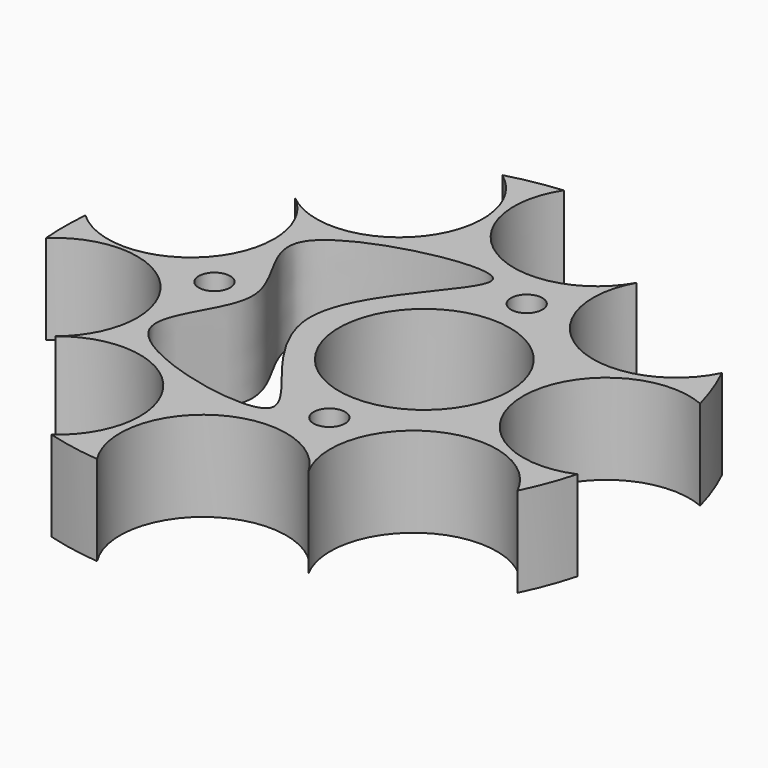
from build123d import *

# Parameters (mm, degrees)
F0_R     = 1.75
F0_R_2   = 9.5
F1_DEPTH = 10


with BuildPart() as f1:
    # F0 (on Top) → F1 (new body)
    with BuildSketch(Plane.XY):
        with BuildLine():
            ThreePointArc((31.353928612, -8.5545987979), (18.4999848113, -0.0237061853), (31.3757496158, 8.4742159547))
            ThreePointArc((31.3757496158, 8.4742159547), (30.4507046637, 11.3580185545), (29.2612387482, 14.1431929536))
            ThreePointArc((29.2612387482, 14.1431929536), (16.6372633011, 10.0158268124), (12.9009909928, 22.7610289132))
            ThreePointArc((12.9009909928, 22.7610289132), (0.046675345, 19.4194010798), (-2.8971318292, 32.3706136359))
            ThreePointArc((-2.8971318292, 32.3706136359), (-5.8977553578, 31.9603892614), (-8.8471652882, 31.2726344647))
            ThreePointArc((-8.8471652882, 31.2726344647), (-6.0434782071, 27.9889108187), (-5.0357213297, 23.7903481709))
            ThreePointArc((-5.0357213297, 23.7903481709), (-10.3432199295, 15.4226015979), (-20.1750040777, 16.6574070724))
            ThreePointArc((-20.1750040777, 16.6574070724), (-17.6965402546, 13.4669673747), (-16.8142868283, 9.5244659761))
            ThreePointArc((-16.8142868283, 9.5244659761), (-22.3815936251, 1.0391686466), (-32.381912941, 2.7679801809))
            ThreePointArc((-32.381912941, 2.7679801809), (-32.4999733171, 0.0416460012), (-32.3889004563, -2.6849817936))
            ThreePointArc((-32.3889004563, -2.6849817936), (-22.3950474365, -0.9770650907), (-16.838610807, -9.4576363939))
            ThreePointArc((-16.838610807, -9.4576363939), (-17.7259230613, -13.410857064), (-20.2176278161, -16.6056472165))
            ThreePointArc((-20.2176278161, -16.6056472165), (-10.3934242287, -15.3909704883), (-5.0966450027, -23.7536581849))
            ThreePointArc((-5.0966450027, -23.7536581849), (-6.10978875, -27.9627791232), (-8.92728264, -31.2498579943))
            ThreePointArc((-8.92728264, -31.2498579943), (-5.9796449934, -31.9451693649), (-2.9800826539, -32.3630824764))
            ThreePointArc((-2.9800826539, -32.3630824764), (-0.0030934102, -19.4194569281), (12.8426160032, -22.7940171899))
            ThreePointArc((12.8426160032, -22.7940171899), (16.6115398174, -10.0584323751), (29.2248960714, -14.2181380503))
            ThreePointArc((29.2248960714, -14.2181380503), (30.4214960056, -11.4360211953), (31.353928612, -8.5545987979))
        make_face()
        with Locations((7.9136770219, -13.7068906766)):
            Circle(F0_R, mode=Mode.SUBTRACT)
        with Locations((-15.8273540437, 0)):
            Circle(F0_R, mode=Mode.SUBTRACT)
        with BuildLine():
            add(Edge.make_bspline(
                [(-5.1913755015, 0), (-5.1913755015, 6.8017390599), (13.8921502508, 20.4717954372), (-22.4625123754, 12.4837485834), (-6.7929208138, 0), (-22.4625123754, -12.4837485834), (13.8921502508, -20.4717954372), (-5.1913755015, -6.8017390599), (-5.1913755015, 0)],
                knots=[0, 0, 0, 0, 0.177937682, 0.3576170923, 0.5, 0.6423829077, 0.822062318, 1, 1, 1, 1], degree=3))
        make_face(mode=Mode.SUBTRACT)
        with Locations((7.5000071177, -0.0007600863)):
            Circle(F0_R_2, mode=Mode.SUBTRACT)
        with Locations((7.9136770219, 13.7068906766)):
            Circle(F0_R, mode=Mode.SUBTRACT)
    extrude(amount=F1_DEPTH)


solid = f1.part
